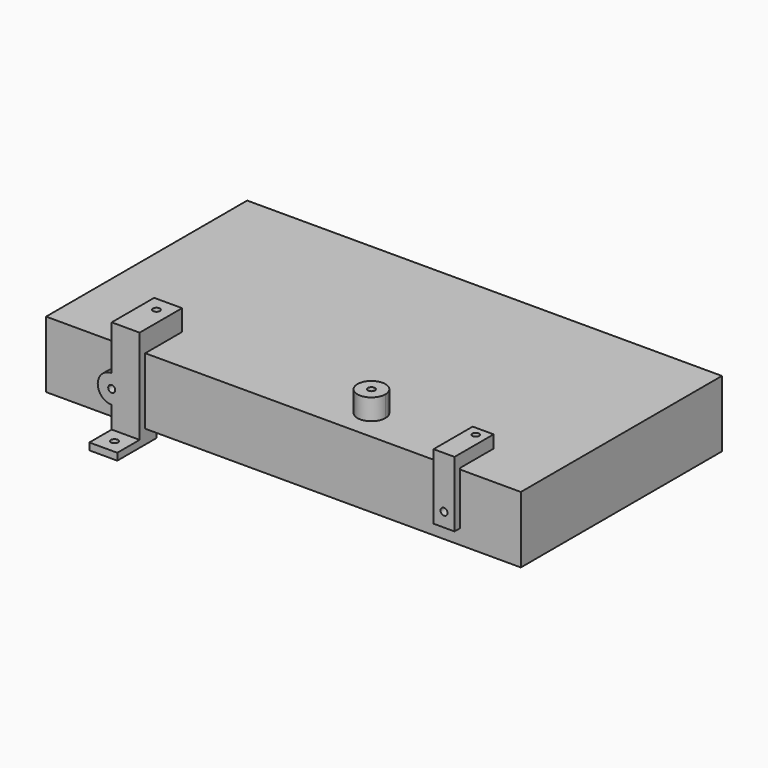
from build123d import *

# Parameters (mm, degrees)
F0_W      = 215.9
F0_H      = 114.3
F1_DEPTH  = 30.226
F4_W      = 12.7
F4_H      = 6.35
F4_H_2    = 9.525
F5_DEPTH  = 3.175
F6_W      = 12.7
F6_H      = 6.35
F7_DEPTH  = 6.35
F6_H_2    = 9.525
F8_DEPTH  = 20.955
F9_W      = 12.7
F9_H      = 3.175
F10_DEPTH = 12.7
F11_R     = 1.5875
F12_DEPTH = 25.4
F13_R     = 1.5875
F14_DEPTH = 25.4
F17_DEPTH = 9.525
F18_W     = 9.525
F18_H     = 23.495
F18_R     = 1.5875
F18_H_2   = 5.715
F18_H_3   = 0.635
F19_DEPTH = 3.175
F20_DEPTH = 19.05
F21_R     = 1.5
F22_DEPTH = 25.4


with BuildPart() as f1:
    # F0 (on Top) → F1 (new body)
    with BuildSketch(Plane.XY):
        Rectangle(F0_W, F0_H)
    extrude(amount=F1_DEPTH)


with BuildPart() as f5:
    # F4 (on face) → F5 (new body)
    with BuildSketch(Plane.XZ.offset(57.15)):
        with Locations((-69.215, -3.175)):
            Rectangle(F4_W, F4_H)
        with BuildLine():
            Line((-75.565, 6.731), (-75.565, 0))
            Line((-75.565, 0), (-62.865, 0))
            Line((-62.865, 0), (-62.865, 30.226))
            Line((-62.865, 30.226), (-75.565, 30.226))
            Line((-75.565, 30.226), (-75.565, 19.431))
            ThreePointArc((-75.565, 19.431), (-71.0748719395, 17.5711280605), (-69.215, 13.081))
            ThreePointArc((-69.215, 13.081), (-71.0748719395, 8.5908719395), (-75.565, 6.731))
        make_face()
        with BuildLine():
            ThreePointArc((-81.915, 13.081), (-80.0551280605, 8.5908719395), (-75.565, 6.731))
            Line((-75.565, 6.731), (-75.565, 11.4935))
            ThreePointArc((-75.565, 11.4935), (-76.6875320151, 11.9584679849), (-77.1525, 13.081))
            Line((-77.1525, 13.081), (-81.915, 13.081))
        make_face()
        with BuildLine():
            Line((-75.565, 11.4935), (-75.565, 6.731))
            ThreePointArc((-75.565, 6.731), (-71.0748719395, 8.5908719395), (-69.215, 13.081))
            ThreePointArc((-69.215, 13.081), (-71.0748719395, 17.5711280605), (-75.565, 19.431))
            Line((-75.565, 19.431), (-75.565, 14.6685))
            ThreePointArc((-75.565, 14.6685), (-74.4424679849, 14.2035320151), (-73.9775, 13.081))
            ThreePointArc((-73.9775, 13.081), (-74.4424679849, 11.9584679849), (-75.565, 11.4935))
        make_face()
        with Locations((-69.215, 34.9885)):
            Rectangle(F4_W, F4_H_2)
        with BuildLine():
            ThreePointArc((-75.565, 19.431), (-80.0551280605, 17.5711280605), (-81.915, 13.081))
            Line((-81.915, 13.081), (-77.1525, 13.081))
            ThreePointArc((-77.1525, 13.081), (-76.6875320151, 14.2035320151), (-75.565, 14.6685))
            Line((-75.565, 14.6685), (-75.565, 19.431))
        make_face()
    extrude(amount=F5_DEPTH)

    # F6 (on face) → F7 (join)
    with BuildSketch(Plane(origin=(0, -57.15, 0), x_dir=(-1, 0, 0), z_dir=(0, 1, 0))):
        with Locations((69.215, -3.175)):
            Rectangle(F6_W, F6_H)
    extrude(amount=F7_DEPTH)

    # F6 (on face) → F8 (join)
    with BuildSketch(Plane(origin=(0, -57.15, 0), x_dir=(-1, 0, 0), z_dir=(0, 1, 0))):
        with Locations((69.215, 34.9885)):
            Rectangle(F6_W, F6_H_2)
    extrude(amount=F8_DEPTH)

    # F9 (on face) → F10 (join)
    with BuildSketch(Plane.XZ.offset(60.325)):
        with Locations((-69.215, -4.7625)):
            Rectangle(F9_W, F9_H)
    extrude(amount=F10_DEPTH)

    # F11 (on face) → F12 (cut)
    with BuildSketch(Plane.XY.offset(-3.175)):
        with Locations((-69.215, -66.675)):
            Circle(F11_R)
    extrude(amount=-F12_DEPTH, mode=Mode.SUBTRACT)

    # F13 (on face) → F14 (cut)
    with BuildSketch(Plane.XY.offset(39.751)):
        with Locations((-69.215, -42.8625)):
            Circle(F13_R)
    extrude(amount=-F14_DEPTH, mode=Mode.SUBTRACT)


with BuildPart() as f17:
    # F16 (on face) → F17 (new body)
    with BuildSketch(Plane.XY.offset(30.226)):
        with BuildLine():
            ThreePointArc((22.225, -42.8625), (28.575, -49.2125), (34.925, -42.8625))
            ThreePointArc((34.925, -42.8625), (33.0651280605, -38.3723719395), (28.575, -36.5125))
            Line((28.575, -36.5125), (28.575, -41.275))
            ThreePointArc((28.575, -41.275), (29.6975320151, -41.7399679849), (30.1625, -42.8625))
            ThreePointArc((30.1625, -42.8625), (28.575, -44.45), (26.9875, -42.8625))
            Line((26.9875, -42.8625), (22.225, -42.8625))
        make_face()
        with BuildLine():
            Line((28.575, -41.275), (28.575, -36.5125))
            ThreePointArc((28.575, -36.5125), (24.0848719395, -38.3723719395), (22.225, -42.8625))
            Line((22.225, -42.8625), (26.9875, -42.8625))
            ThreePointArc((26.9875, -42.8625), (27.4524679849, -41.7399679849), (28.575, -41.275))
        make_face()
    extrude(amount=F17_DEPTH)


with BuildPart() as f19:
    # F18 (on face) → F19 (new body)
    with BuildSketch(Plane.XZ.offset(57.15)):
        with Locations((75.565, 18.4785)):
            Rectangle(F18_W, F18_H)
        with Locations((75.565, 13.081)):
            Circle(F18_R, mode=Mode.SUBTRACT)
        with Locations((75.565, 33.7185)):
            Rectangle(F18_W, F18_H_2)
        with Locations((75.565, 30.5435)):
            Rectangle(F18_W, F18_H_3)
    extrude(amount=F19_DEPTH)

    # F18 (on face) → F20 (join)
    with BuildSketch(Plane.XZ.offset(57.15)):
        with Locations((75.565, 33.7185)):
            Rectangle(F18_W, F18_H_2)
    extrude(amount=-F20_DEPTH)

    # F21 (on face) → F22 (cut)
    with BuildSketch(Plane.XY.offset(36.576)):
        with Locations((75.565, -42.2774255276)):
            Circle(F21_R)
    extrude(amount=-F22_DEPTH, mode=Mode.SUBTRACT)


solid = Compound([f1.part, f5.part, f17.part, f19.part])
